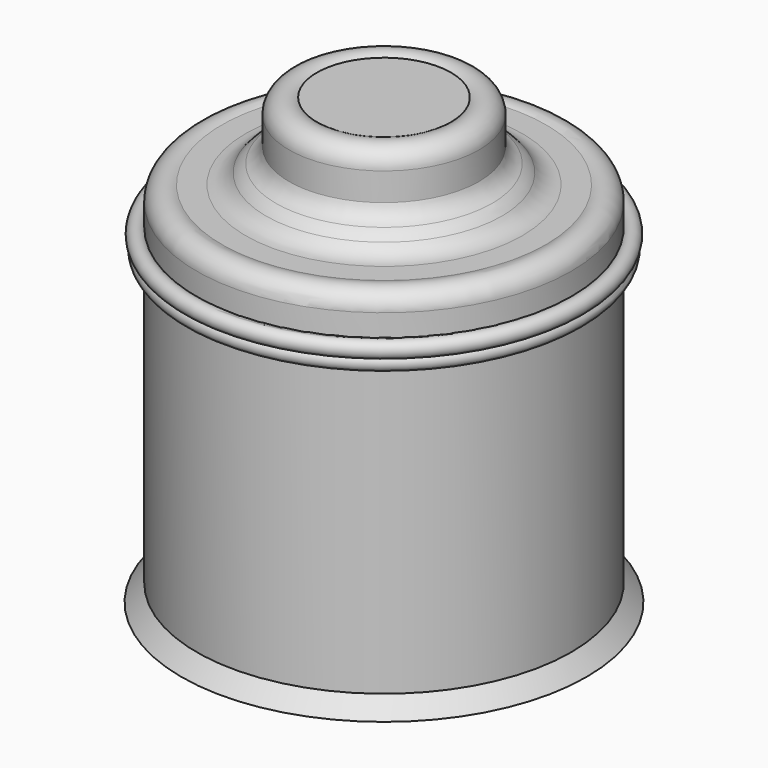
from build123d import *

# Parameters (mm, degrees)
F2_R = 5.08


with BuildPart() as f1:
    # F0 (on Front) → F1 (revolve)
    with BuildSketch(Plane.XZ):
        with BuildLine():
            Line((25.6270375103, -20.7102242857), (25.6270375103, 40.9734621644))
            ThreePointArc((25.6270375103, 40.9734621644), (27.8491666489, 41.1532383904), (27.9331301745, 43.3810461754))
            ThreePointArc((27.9331301745, 43.3810461754), (28.2766730596, 46.0084963098), (25.6270375103, 46.039275825))
            Line((25.6270375103, 46.039275825), (25.6270375103, 50.8070923388))
            ThreePointArc((25.6270375103, 50.8070923388), (23.8643122828, 53.9501330087), (20.2632397413, 54.0849715471))
            Line((20.2632397413, 54.0849715471), (15.1974307373, 54.0849715471))
            ThreePointArc((15.1974307373, 54.0849715471), (12.0970574014, 55.0689926556), (10.1316217333, 57.6608404517))
            ThreePointArc((10.1316217333, 57.6608404517), (7.4985266441, 58.8104034839), (5.9597794898, 61.236705631))
            Line((5.9597794898, 61.236705631), (5.9597794898, 67.1964809299))
            ThreePointArc((5.9597794898, 67.1964809299), (3.9489469256, 70.5973425578), (0, 70.4743564129))
            Line((0, 70.4743564129), (-14.3034653738, 70.4743564129))
            Line((-14.3034653738, 70.4743564129), (-14.3034653738, -24.286089465))
            Line((-14.3034653738, -24.286089465), (28.904914856, -24.286089465))
            Line((28.904914856, -24.286089465), (25.6270375103, -20.7102242857))
        make_face()
        with BuildLine():
            ThreePointArc((25.6270375103, 43.6553657055), (26.8351751992, 43.9813365596), (27.9331301745, 43.3810461754))
            ThreePointArc((27.9331301745, 43.3810461754), (26.7288801976, 43.0877577338), (25.6270375103, 43.6553657055))
        make_face(mode=Mode.SUBTRACT)
        with BuildLine():
            ThreePointArc((25.6270375103, 43.6553657055), (26.7288801976, 43.0877577338), (27.9331301745, 43.3810461754))
            ThreePointArc((27.9331301745, 43.3810461754), (26.8351751992, 43.9813365596), (25.6270375103, 43.6553657055))
        make_face()
    revolve(axis=Axis((-14.3034653738, 0, 23.0941334739), (0, 0, -1)))

    # F2
    f2_edges = [f1.edges().sort_by_distance(p)[0] for p in [
        (-38.738552, 0, 57.66084),
    ]]
    fillet(f2_edges, radius=F2_R)


solid = f1.part
